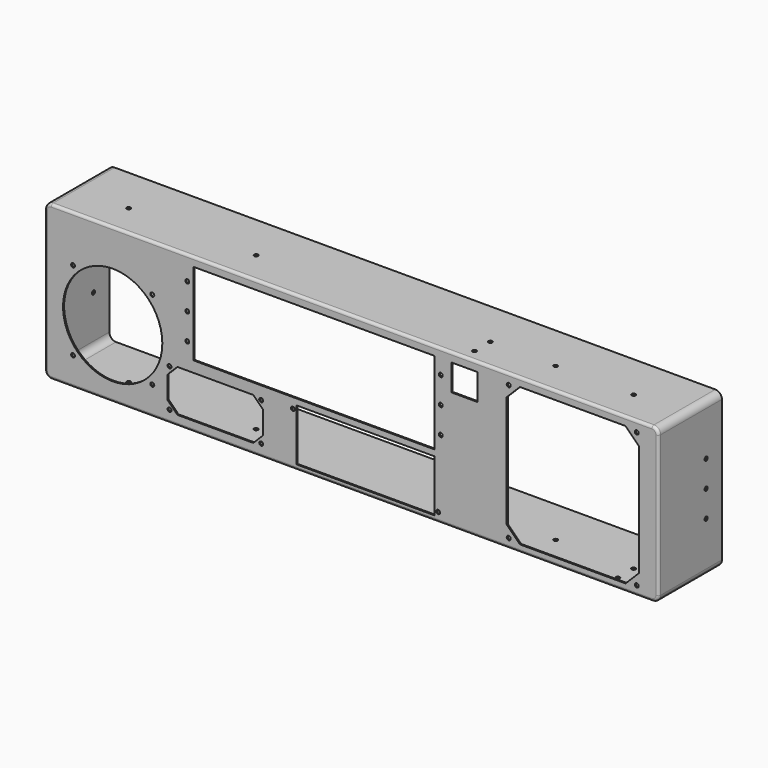
from build123d import *

# Parameters (mm, degrees)
F0_W              = 465
F0_H              = 117
F1_DEPTH          = 60
F2_T              = -1
F3_W              = 20
F3_H              = 20
F3_R              = 1.5
F3_R_2            = 37.6
F3_W_2            = 182.4
F3_H_2            = 62.4
F3_W_3            = 104.4
F3_H_3            = 39.4
F4_DEPTH          = 25
F5_R              = 1.5
F6_DEPTH          = 500
F10_R             = 1.5
F11_DEPTH         = 2
F11_COPIES1_COUNT = 2
F11_COPIES1_PITCH = 60.876925
F11_COPIES2_COUNT = 2
F11_COPIES2_PITCH = 286.393087
F11_COPIES3_COUNT = 2
F11_COPIES3_PITCH = 382.794005
F11_COPIES4_COUNT = 2
F11_COPIES4_PITCH = 116.965807
F11_COPIES5_COUNT = 2
F11_COPIES5_PITCH = 131.003817
F11_COPIES6_COUNT = 2
F11_COPIES6_PITCH = 308.993527
F11_COPIES7_COUNT = 2
F11_COPIES7_PITCH = 399.984062
F11_COPIES8_COUNT = 2
F11_COPIES8_PITCH = 158.834033
F11_COPIES9_COUNT = 2
F11_COPIES9_PITCH = 159.540747
F12_R             = 5
F13_R             = 2


# Not quite as in the source:
# - a feature of the source that left no trace in its solid (it failed there, or was rolled back) is left out
# - a pattern or mirror of a feature is missing from the dataset's text; its kind, count and spacing are read off the source's solid


with BuildPart() as f1:
    # F0 (on Front) → F1 (new body)
    with BuildSketch(Plane.XZ):
        with Locations((-12.6529467106, 27.1878533959)):
            Rectangle(F0_W, F0_H)
    extrude(amount=F1_DEPTH)

    # F2
    f2_openings = [f1.faces().sort_by_distance(p)[0] for p in [
        (-12.652947, 0, 27.187853),
    ]]
    offset(amount=F2_T, openings=f2_openings)

    # F3 (on face) → F4 (cut)
    with BuildSketch(Plane.XZ.offset(60)):
        with Locations((72.8470532894, 68.6878533959)):
            Rectangle(F3_W, F3_H)
        Polygon((194.8470532894, 79.1878533959), (114.8470532894, 79.1878533959), (104.8470532894, 69.1878533959), (104.8470532894, -15.8121466041), (114.8470532894, -25.8121466041), (194.8470532894, -25.8121466041), (204.8470532894, -15.8121466041), (204.8470532894, 69.1878533959), align=None)
        with Locations((54.8470532894, 67.6878533959)):
            Circle(F3_R)
        with Locations((54.8470532894, 47.6878533959)):
            Circle(F3_R)
        with Locations((54.8470532894, 27.6878533959)):
            Circle(F3_R)
        with Locations((106.3470532894, 77.6878533959)):
            Circle(F3_R)
        Polygon((-87.1529467106, 8.1878533959), (-144.6529467106, 8.1878533959), (-152.1529467106, 0.6878533959), (-152.1529467106, -16.3121466041), (-144.6529467106, -23.8121466041), (-87.1529467106, -23.8121466041), (-79.6529467106, -16.3121466041), (-79.6529467106, 0.6878533959), align=None)
        with Locations((-193.6529467106, 20.1878533959)):
            Circle(F3_R_2)
        with Locations((-137.1529467106, 67.6878533959)):
            Circle(F3_R)
        with Locations((-137.1529467106, 47.6878533959)):
            Circle(F3_R)
        with Locations((-137.1529467106, 27.6878533959)):
            Circle(F3_R)
        with Locations((-223.6529467106, 50.1878533959)):
            Circle(F3_R)
        with Locations((-223.6529467106, -9.8121466041)):
            Circle(F3_R)
        with Locations((-163.6529467106, -9.8121466041)):
            Circle(F3_R)
        with Locations((-163.6529467106, 50.1878533959)):
            Circle(F3_R)
        with Locations((-57.1529467106, 8.6878533959)):
            Circle(F3_R)
        with Locations((52.8470532894, -24.3121466041)):
            Circle(F3_R)
        with Locations((-150.6529467106, 6.6878533959)):
            Circle(F3_R)
        with Locations((-81.1529467106, 6.6878533959)):
            Circle(F3_R)
        with Locations((-150.6529467106, -22.3121466041)):
            Circle(F3_R)
        with Locations((-81.1529467106, -22.3121466041)):
            Circle(F3_R)
        with Locations((203.3470532894, 77.6878533959)):
            Circle(F3_R)
        with Locations((106.3470532894, -24.3121466041)):
            Circle(F3_R)
        with Locations((203.3470532894, -24.3121466041)):
            Circle(F3_R)
        with Locations((-41.1529467106, 47.6878533959)):
            Rectangle(F3_W_2, F3_H_2)
        with Locations((-2.1529467106, -7.8121466041)):
            Rectangle(F3_W_3, F3_H_3)
    extrude(amount=-F4_DEPTH, mode=Mode.SUBTRACT)

    # F5 (on face) → F6 (cut)
    with BuildSketch(Plane(origin=(-245.1529467106, 0, 0), x_dir=(0, -1, 0), z_dir=(-1, 0, 0))):
        with Locations((15, 47.1878533959)):
            Circle(F5_R)
        with Locations((15, 7.1878533959)):
            Circle(F5_R)
        with Locations((15, 27.1878533959)):
            Circle(F5_R)
    extrude(amount=-F6_DEPTH, mode=Mode.SUBTRACT)

    # F10 (on face) → F11 (cut)
    with BuildSketch(Plane(origin=(0, 0, -31.3121466041), x_dir=(1, 0, 0), z_dir=(0, 0, -1))):
        with Locations((181.3470532894, 50.5)):
            Circle(F10_R)
    f11 = extrude(amount=-F11_DEPTH, mode=Mode.SUBTRACT)

    # F11_copies: F11 across plane
    add(f11.mirror(Plane.ZX.offset(-43)), mode=Mode.SUBTRACT)

    # F11_copies1: F11 ×2
    with Locations(*[Vector(-0.9691685311, 0.2463987791, 0) * (i * F11_COPIES1_PITCH) for i in range(1, F11_COPIES1_COUNT)]):
        add(f11, mode=Mode.SUBTRACT)

    # F11_copies2: F11 ×2
    with Locations(*[Vector(-0.9986274581, 0.052375566, 0) * (i * F11_COPIES2_PITCH) for i in range(1, F11_COPIES2_COUNT)]):
        add(f11, mode=Mode.SUBTRACT)

    # F11_copies3: F11 ×2
    with Locations(*[Vector(-0.9992319507, 0.0391855667, 0) * (i * F11_COPIES3_PITCH) for i in range(1, F11_COPIES3_COUNT)]):
        add(f11, mode=Mode.SUBTRACT)

    # F11_copies4: F11 ×2
    with Locations(*[Vector(0, 0.1282426069, 0.9917428264) * (i * F11_COPIES4_PITCH) for i in range(1, F11_COPIES4_COUNT)]):
        add(f11, mode=Mode.SUBTRACT)

    # F11_copies5: F11 ×2
    with Locations(*[Vector(-0.4503685577, 0.1145004808, 0.8854703847) * (i * F11_COPIES5_PITCH) for i in range(1, F11_COPIES5_COUNT)]):
        add(f11, mode=Mode.SUBTRACT)

    # F11_copies6: F11 ×2
    with Locations(*[Vector(-0.9255857311, 0.0485447062, 0.3754123944) * (i * F11_COPIES6_PITCH) for i in range(1, F11_COPIES6_COUNT)]):
        add(f11, mode=Mode.SUBTRACT)

    # F11_copies7: F11 ×2
    with Locations(*[Vector(-0.9562881029, 0.0375014942, 0.2900115554) * (i * F11_COPIES7_PITCH) for i in range(1, F11_COPIES7_COUNT)]):
        add(f11, mode=Mode.SUBTRACT)

    # F11_copies8: F11 ×2
    with Locations(*[Vector(-0.6831029725, 0, 0.730322072) * (i * F11_COPIES8_PITCH) for i in range(1, F11_COPIES8_COUNT)]):
        add(f11, mode=Mode.SUBTRACT)

    # F11_copies9: F11 ×2
    with Locations(*[Vector(-0.6800770458, 0.0940198681, 0.7270869798) * (i * F11_COPIES9_PITCH) for i in range(1, F11_COPIES9_COUNT)]):
        add(f11, mode=Mode.SUBTRACT)

    # F12
    f12_edges = [f1.edges().sort_by_distance(p)[0] for p in [
        (-245.152947, -30, 85.687853),
        (219.847053, -30, 85.687853),
        (219.847053, -30, -31.312147),
        (-245.152947, -30, -31.312147),
        (-244.152947, -29.5, 84.687853),
        (-244.152947, -29.5, -30.312147),
        (218.847053, -29.5, -30.312147),
        (218.847053, -29.5, 84.687853),
    ]]
    fillet(f12_edges, radius=F12_R)

    # F13
    f13_edges = [f1.edges().sort_by_distance(p)[0] for p in [
        (218.382587, -60, 84.223387),
        (-12.652947, -59, 84.687853),
        (-12.652947, -60, -31.312147),
        (-243.688481, -60, -29.847681),
        (218.382587, -60, -29.847681),
        (-245.152947, -60, 27.187853),
        (219.847053, -60, 27.187853),
        (-243.688481, -60, 84.223387),
        (-12.652947, -60, 85.687853),
        (-12.652947, -59, -30.312147),
        (-242.688481, -59, -28.847681),
        (217.382587, -59, -28.847681),
        (-244.152947, -59, 27.187853),
        (218.847053, -59, 27.187853),
        (-242.688481, -59, 83.223387),
        (217.382587, -59, 83.223387),
    ]]
    fillet(f13_edges, radius=F13_R)


solid = f1.part
